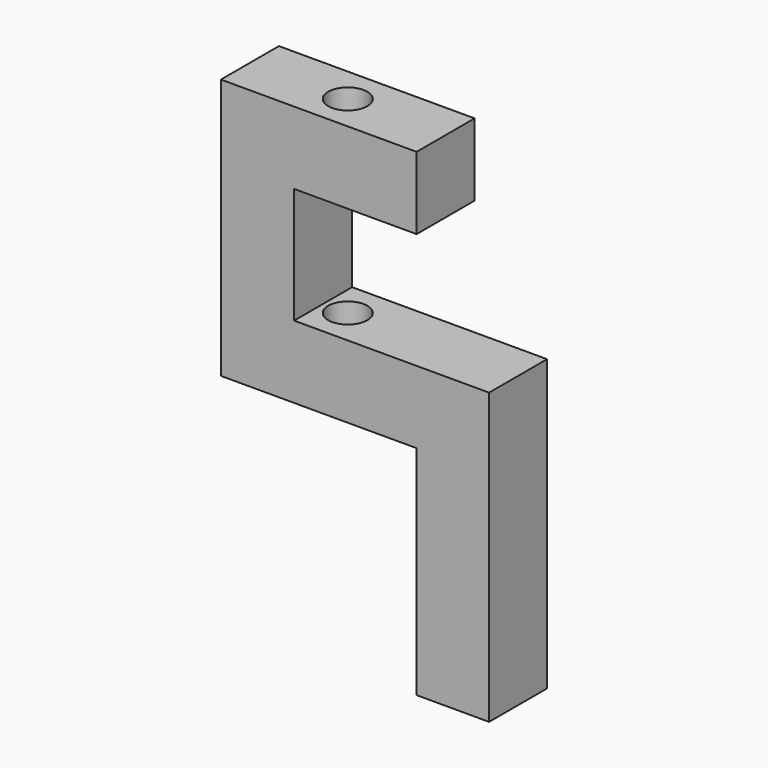
from build123d import *

# Parameters (mm, degrees)
F2_DEPTH = 10
F4_D     = 5.4


# Not quite as in the source:
# - a feature names something its author has since deleted; it is built from what else it names


with BuildPart() as f2:
    # F1 (on Front) → F2 (new body)
    with BuildSketch(Plane.XZ):
        Polygon((-36.8737237304, 13.780983012), (-63.8737237304, 13.780983012), (-63.8737237304, -22.219016988), (-36.8737237304, -22.219016988), (-36.8737237304, -52.219016988), (-26.8737237304, -52.219016988), (-26.8737237304, -12.219016988), (-36.8737237304, -12.219016988), (-53.7737237304, -12.219016988), (-53.7737237304, 3.780983012), (-36.8737237304, 3.780983012), align=None)
    extrude(amount=F2_DEPTH)

    # F4 (through all)
    with Locations(Plane.XY.offset(13.780983012)):
        with Locations((-50.3737237304, -5)):
            Hole(F4_D / 2)


solid = f2.part
